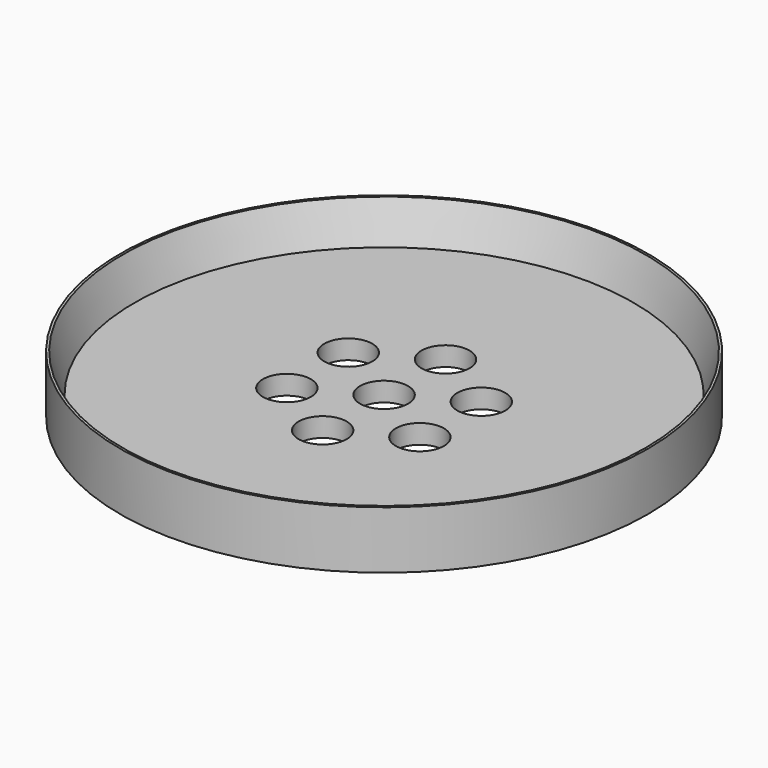
from build123d import *

# Parameters (mm, degrees)
F0_R     = 26
F0_R_2   = 12
F0_R_3   = 2.5
F1_DEPTH = 2
F0_R_4   = 27.5
F2_DEPTH = 6
F3_SIZE2 = 1.24999
F3_SIZE  = 3.99999


# Not quite as in the source:
# - a fillet or chamfer is up to 0.001 mm smaller than in the source, because OpenCascade refuses the exact size


with BuildPart() as f1:
    # F0 (on Top) → F1 (new body)
    with BuildSketch(Plane.XY):
        Circle(F0_R)
        Circle(F0_R_2, mode=Mode.SUBTRACT)
        Circle(F0_R_2)
        with Locations((-6.9282032303, -4)):
            Circle(F0_R_3, mode=Mode.SUBTRACT)
        with Locations((0, -8)):
            Circle(F0_R_3, mode=Mode.SUBTRACT)
        with Locations((6.9282032303, -4)):
            Circle(F0_R_3, mode=Mode.SUBTRACT)
        with Locations((-6.9282032303, 4)):
            Circle(F0_R_3, mode=Mode.SUBTRACT)
        Circle(F0_R_3, mode=Mode.SUBTRACT)
        with Locations((6.9282032303, 4)):
            Circle(F0_R_3, mode=Mode.SUBTRACT)
        with Locations((0, 8)):
            Circle(F0_R_3, mode=Mode.SUBTRACT)
    extrude(amount=F1_DEPTH)

    # F0 (on Top) → F2 (join)
    with BuildSketch(Plane.XY):
        Circle(F0_R_4)
        Circle(F0_R, mode=Mode.SUBTRACT)
    extrude(amount=F2_DEPTH)

    # F3 (size 4 and 1.25 in the source; OpenCascade refuses exactly that, so slightly less here)
    f3_edges = [f1.edges().sort_by_distance(p)[0] for p in [
        (-26, 0, 6),
    ]]
    f3_side = f1.faces().sort_by_distance((-26, 0, 4))[0]
    chamfer(f3_edges, length=F3_SIZE, length2=F3_SIZE2, reference=f3_side)


solid = f1.part
